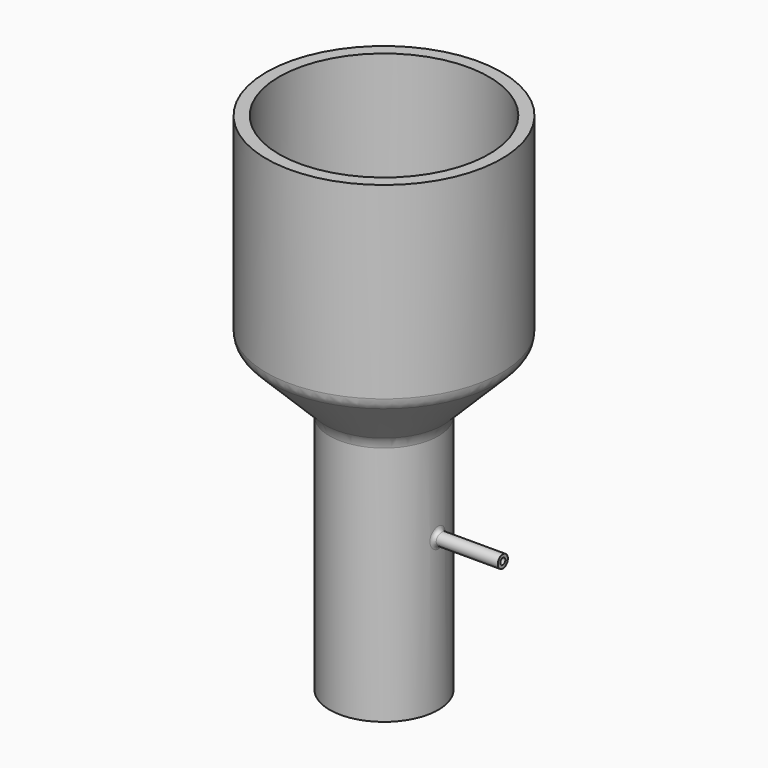
from build123d import *

# Parameters (mm, degrees)
F2_R     = 1.25
F4_R     = 0.25
F5_DEPTH = 9.4
F6_R     = 0.5
F6_R_2   = 0.25
F8_R     = 0.3


with BuildPart() as f1:
    # F0 (on Front) → F1 (revolve)
    with BuildSketch(Plane.XZ):
        Polygon((-4.3, 0), (-3.3, 0), (-3.3, 20), (-8.3, 25), (-8.3, 40), (-9.3, 40), (-9.3, 24.5857864376), (-4.3, 19.5857864376), align=None)
    revolve(axis=Axis((0, 0, 9.394146502), (0, 0, 1)))

    # F2
    f2_edges = [f1.edges().sort_by_distance(p)[0] for p in [
        (9.3, 0, 24.585786),
        (4.3, 0, 19.585786),
        (8.3, 0, 25),
        (3.3, 0, 20),
    ]]
    fillet(f2_edges, radius=F2_R)

    # F4 (on Right) → F5 (cut, through all)
    with BuildSketch(Plane.YZ):
        with Locations((0, 12)):
            Circle(F4_R)
    extrude(amount=F5_DEPTH, mode=Mode.SUBTRACT)

    # F6 (on offset) → F7 (join, up to the next surface of F1)
    with BuildSketch(Plane.YZ.offset(9.4)):
        with Locations((0, 12)):
            Circle(F6_R)
        with Locations((0, 12)):
            Circle(F6_R_2, mode=Mode.SUBTRACT)
    extrude(until=Until.NEXT, dir=(-1, 0, 0))

    # F8
    f8_edges = [f1.edges().sort_by_distance(p)[0] for p in [
        (4.270831, -0.5, 12),
        (3.290517, -0.25, 12),
    ]]
    fillet(f8_edges, radius=F8_R)


solid = f1.part
